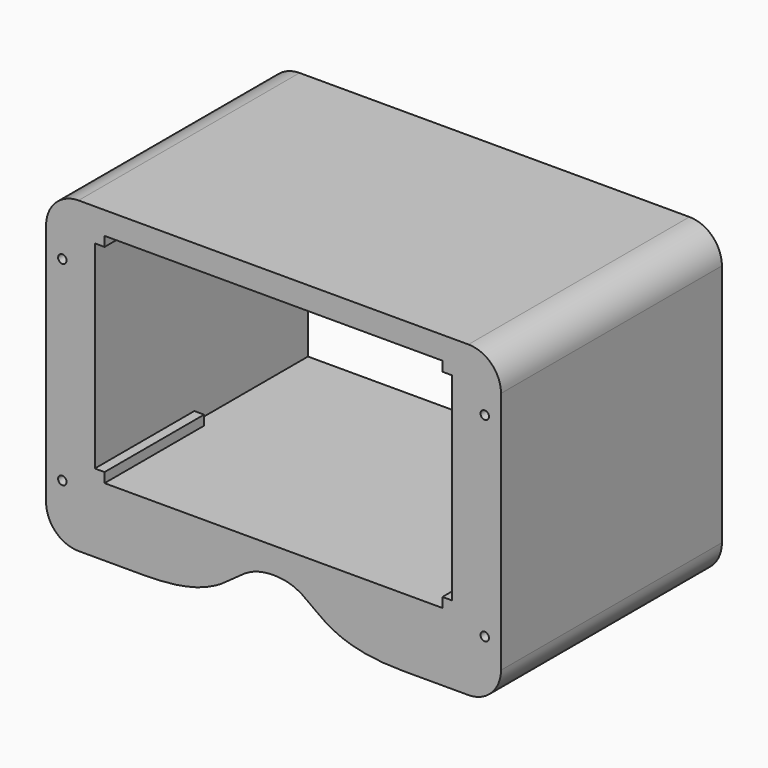
from build123d import *

# Parameters (mm, degrees)
F0_W      = 140
F0_H      = 170
F1_DEPTH  = 95
F2_W      = 110
F2_H      = 67
F3_DEPTH  = 170.001
F5_DEPTH  = 88
F7_DEPTH  = 95.001
F8_R      = 10
F10_DEPTH = 170.001
F11_W     = 121
F11_H     = 76
F11_W_2   = 110
F11_H_2   = 67
F12_DEPTH = 3
F13_W     = 3
F13_H     = 90
F14_DEPTH = 3
F15_W     = 3
F15_H     = 90
F16_DEPTH = 3
F17_R     = 1.3
F18_DEPTH = 100
F19_R     = 3.1
F20_DEPTH = 75
F21_W     = 145
F21_H     = 89.208022
F22_DEPTH = 95.001


with BuildPart() as f1:
    # F0 (on Top) → F1 (new body)
    with BuildSketch(Plane.XY):
        Rectangle(F0_W, F0_H)
    extrude(amount=F1_DEPTH)

    # F2 (on face) → F3 (cut, through all)
    with BuildSketch(Plane.XZ.offset(85)):
        with Locations((0, 54.5)):
            Rectangle(F2_W, F2_H)
    extrude(amount=-F3_DEPTH, mode=Mode.SUBTRACT)

    # F4 (on face) → F5 (cut)
    with BuildSketch(Plane(origin=(0, 0, 0), x_dir=(1, 0, 0), z_dir=(0, 0, -1))):
        with BuildLine():
            add(Edge.make_bspline(
                [(0, 15), (-7.79441, 15), (-19.466411, 48.056936), (-30.975012, 59.107625), (-57.856268, 61.12551), (-68.258241, 85)],
                knots=[0, 0, 0, 0, 0.355883, 0.597297, 1, 1, 1, 1], degree=3))
            add(Edge.make_bspline(
                [(0, 15), (7.79441, 15), (19.466411, 48.056936), (30.975012, 59.107625), (57.856268, 61.12551), (68.258241, 85)],
                knots=[0, 0, 0, 0, 0.355883, 0.597297, 1, 1, 1, 1], degree=3))
            Line((68.258241, 85), (-68.258241, 85))
        make_face()
    extrude(amount=-F5_DEPTH, mode=Mode.SUBTRACT)

    # F6 (on face) → F7 (cut, through all)
    with BuildSketch(Plane.XY.offset(95)):
        with BuildLine():
            add(Edge.make_bspline(
                [(0, -55), (25.389496, -55), (47.041007, -60.614282), (62.843867, -75.413413), (68.355819, -85)],
                knots=[0, 0, 0, 0, 0.564508, 1, 1, 1, 1], degree=3))
            add(Edge.make_bspline(
                [(0, -55), (-25.389496, -55), (-47.041007, -60.614282), (-62.843867, -75.413413), (-68.355819, -85)],
                knots=[0, 0, 0, 0, 0.564508, 1, 1, 1, 1], degree=3))
            Line((-68.355819, -85), (68.355819, -85))
        make_face()
    extrude(amount=-F7_DEPTH, mode=Mode.SUBTRACT)

    # F8
    f8_edges = [f1.edges().sort_by_distance(p)[0] for p in [
        (70, 0, 95),
        (70, 0, 0),
        (-70, 0, 0),
        (-70, 0, 95),
    ]]
    fillet(f8_edges, radius=F8_R)

    # F9 (on face) → F10 (cut, through all)
    with BuildSketch(Plane(origin=(0, 85, 0), x_dir=(-1, 0, 0), z_dir=(0, 1, 0))):
        with BuildLine():
            add(Edge.make_bspline(
                [(0, 13), (14.179069, 13), (11.016984, 0), (40, 0)],
                knots=[0, 0, 0, 0, 42.059482, 42.059482, 42.059482, 42.059482], degree=3))
            add(Edge.make_bspline(
                [(0, 13), (-14.179069, 13), (-11.016984, 0), (-40, 0)],
                knots=[0, 0, 0, 0, 42.059482, 42.059482, 42.059482, 42.059482], degree=3))
            Line((-40, 0), (40, 0))
        make_face()
    extrude(amount=-F10_DEPTH, mode=Mode.SUBTRACT)

    # F11 (on face) → F12 (cut)
    with BuildSketch(Plane(origin=(0, 85, 0), x_dir=(-1, 0, 0), z_dir=(0, 1, 0))):
        with Locations((0, 52)):
            Rectangle(F11_W, F11_H)
        with Locations((0, 54.5)):
            Rectangle(F11_W_2, F11_H_2, mode=Mode.SUBTRACT)
    extrude(amount=-F12_DEPTH, mode=Mode.SUBTRACT)

    # F13 (on face) → F14 (join)
    with BuildSketch(Plane.XY.offset(21)):
        with Locations((-53.5, -6.706829)):
            Rectangle(F13_W, F13_H)
        with Locations((53.5, -6.706829)):
            Rectangle(F13_W, F13_H)
    extrude(amount=F14_DEPTH)

    # F15 (on face) → F16 (join)
    with BuildSketch(Plane(origin=(0, 0, 88), x_dir=(1, 0, 0), z_dir=(0, 0, -1))):
        with Locations((53.5, 6.706829)):
            Rectangle(F15_W, F15_H)
        with Locations((-53.5, 6.706829)):
            Rectangle(F15_W, F15_H)
    extrude(amount=F16_DEPTH)

    # F17 (on face) → F18 (cut)
    with BuildSketch(Plane(origin=(0, 85, 0), x_dir=(-1, 0, 0), z_dir=(0, 1, 0))):
        with Locations((65, 77.5)):
            Circle(F17_R)
        with Locations((65, 17.5)):
            Circle(F17_R)
        with Locations((-65, 77.5)):
            Circle(F17_R)
        with Locations((-65, 17.5)):
            Circle(F17_R)
    extrude(amount=-F18_DEPTH, mode=Mode.SUBTRACT)

    # F19 (on face) → F20 (cut)
    with BuildSketch(Plane(origin=(0, 85, 0), x_dir=(-1, 0, 0), z_dir=(0, 1, 0))):
        with Locations((65, 77.5)):
            Circle(F19_R)
        with Locations((65, 17.5)):
            Circle(F19_R)
        with Locations((-65, 77.5)):
            Circle(F19_R)
        with Locations((-65, 17.5)):
            Circle(F19_R)
    extrude(amount=-F20_DEPTH, mode=Mode.SUBTRACT)

    # F21 (on face) → F22 (cut, through all)
    with BuildSketch(Plane.XY.offset(95)):
        with Locations((-0.091513, -44.604011)):
            Rectangle(F21_W, F21_H)
    extrude(amount=-F22_DEPTH, mode=Mode.SUBTRACT)


solid = f1.part
